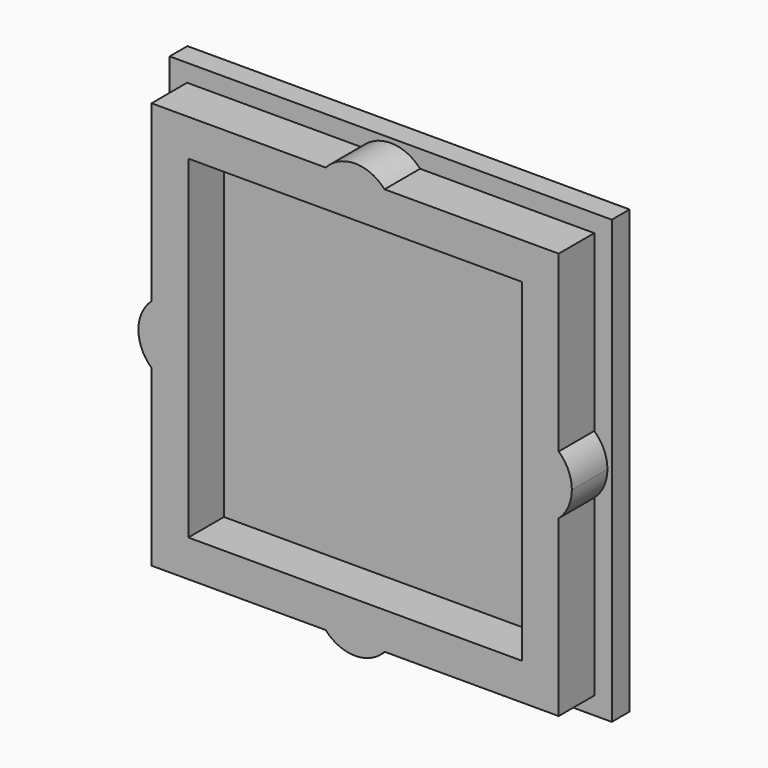
from build123d import *

# Parameters (mm, degrees)
F1_DEPTH = 7.62
F0_W     = 50.5
F0_H     = 50.5
F2_DEPTH = 2.54
F3_W     = 38.1
F3_H     = 38.1
F4_DEPTH = 5.08


# Not quite as in the source:
# - a feature names something its author has since deleted; it is built from what else it names


with BuildPart() as f1:
    # F0 (on Front) → F1 (new body)
    with BuildSketch(Plane.XZ):
        with BuildLine():
            Line((-3.3566042603, 23.25), (-23.25, 23.25))
            Line((-23.25, 23.25), (-23.25, 3.3541019662))
            ThreePointArc((-23.25, 3.3541019662), (-18.4128826929, 4.1079191813), (-15.75, 0))
            ThreePointArc((-15.75, 0), (-18.4128826929, -4.1079191813), (-23.25, -3.3541019662))
            Line((-23.25, -3.3541019662), (-23.25, -23.25))
            Line((-23.25, -23.25), (-3.3566042603, -23.25))
            ThreePointArc((-3.3566042603, -23.25), (-1.6039452654, -16.0483547827), (4.5, -20.2528))
            ThreePointArc((4.5, -20.2528), (4.2044452173, -21.8567452654), (3.3566042603, -23.25))
            Line((3.3566042603, -23.25), (23.25, -23.25))
            Line((23.25, -23.25), (23.25, -3.3566042603))
            ThreePointArc((23.25, -3.3566042603), (15.7528, 0), (23.25, 3.3566042603))
            Line((23.25, 3.3566042603), (23.25, 23.25))
            Line((23.25, 23.25), (3.3566042603, 23.25))
            ThreePointArc((3.3566042603, 23.25), (4.2044452173, 21.8567452654), (4.5, 20.2528))
            ThreePointArc((4.5, 20.2528), (-1.6039452654, 16.0483547827), (-3.3566042603, 23.25))
        make_face()
        with BuildLine():
            ThreePointArc((3.3566042603, 23.25), (0, 24.7528), (-3.3566042603, 23.25))
            Line((-3.3566042603, 23.25), (3.3566042603, 23.25))
        make_face()
        with BuildLine():
            Line((3.3566042603, 23.25), (-3.3566042603, 23.25))
            ThreePointArc((-3.3566042603, 23.25), (-1.6039452654, 16.0483547827), (4.5, 20.2528))
            ThreePointArc((4.5, 20.2528), (4.2044452173, 21.8567452654), (3.3566042603, 23.25))
        make_face()
        with BuildLine():
            ThreePointArc((-15.75, 0), (-18.4128826929, 4.1079191813), (-23.25, 3.3541019662))
            Line((-23.25, 3.3541019662), (-23.25, -3.3541019662))
            ThreePointArc((-23.25, -3.3541019662), (-18.4128826929, -4.1079191813), (-15.75, 0))
        make_face()
        with BuildLine():
            Line((-23.25, -3.3541019662), (-23.25, 3.3541019662))
            ThreePointArc((-23.25, 3.3541019662), (-24.75, 0), (-23.25, -3.3541019662))
        make_face()
        with BuildLine():
            ThreePointArc((4.5, -20.2528), (-1.6039452654, -16.0483547827), (-3.3566042603, -23.25))
            Line((-3.3566042603, -23.25), (3.3566042603, -23.25))
            ThreePointArc((3.3566042603, -23.25), (4.2044452173, -21.8567452654), (4.5, -20.2528))
        make_face()
        with BuildLine():
            Line((3.3566042603, -23.25), (-3.3566042603, -23.25))
            ThreePointArc((-3.3566042603, -23.25), (0, -24.7528), (3.3566042603, -23.25))
        make_face()
        with BuildLine():
            Line((23.25, -3.3566042603), (23.25, 3.3566042603))
            ThreePointArc((23.25, 3.3566042603), (15.7528, 0), (23.25, -3.3566042603))
        make_face()
        with BuildLine():
            ThreePointArc((24.7528, 0), (24.3599522981, 1.8388311505), (23.25, 3.3566042603))
            Line((23.25, 3.3566042603), (23.25, -3.3566042603))
            ThreePointArc((23.25, -3.3566042603), (24.3599522981, -1.8388311505), (24.7528, 0))
        make_face()
    extrude(amount=F1_DEPTH)

    # F0 (on Front) → F2 (join)
    with BuildSketch(Plane.XZ):
        Rectangle(F0_W, F0_H)
        with BuildLine():
            Line((-23.25, 3.3541019662), (-23.25, 23.25))
            Line((-23.25, 23.25), (-3.3566042603, 23.25))
            ThreePointArc((-3.3566042603, 23.25), (0, 24.7528), (3.3566042603, 23.25))
            Line((3.3566042603, 23.25), (23.25, 23.25))
            Line((23.25, 23.25), (23.25, 3.3566042603))
            ThreePointArc((23.25, 3.3566042603), (24.3599522981, 1.8388311505), (24.7528, 0))
            ThreePointArc((24.7528, 0), (24.3599522981, -1.8388311505), (23.25, -3.3566042603))
            Line((23.25, -3.3566042603), (23.25, -23.25))
            Line((23.25, -23.25), (3.3566042603, -23.25))
            ThreePointArc((3.3566042603, -23.25), (0, -24.7528), (-3.3566042603, -23.25))
            Line((-3.3566042603, -23.25), (-23.25, -23.25))
            Line((-23.25, -23.25), (-23.25, -3.3541019662))
            ThreePointArc((-23.25, -3.3541019662), (-24.75, 0), (-23.25, 3.3541019662))
        make_face(mode=Mode.SUBTRACT)
    extrude(amount=F2_DEPTH)

    # F3 (on face) → F4 (cut)
    with BuildSketch(Plane.XZ.offset(7.62)):
        Rectangle(F3_W, F3_H)
    extrude(amount=-F4_DEPTH, mode=Mode.SUBTRACT)


solid = f1.part
